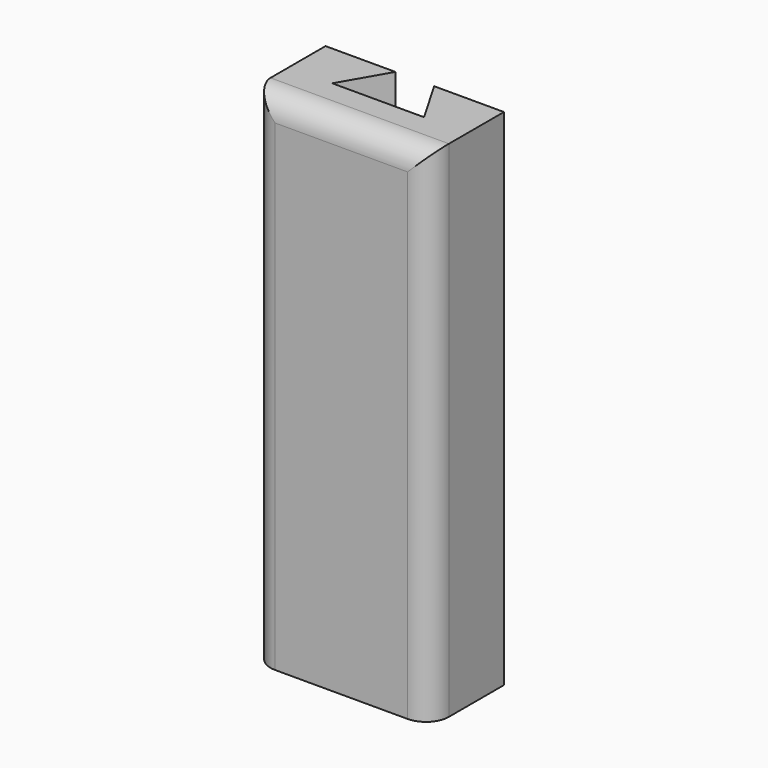
from build123d import *

# Parameters (mm, degrees)
F1_DEPTH    = 279.4
F2_T1_DEPTH = 136.906


# Not quite as in the source:
# - a fillet or chamfer that OpenCascade refuses, or shapes differently, is made with other operations: its cross-section is extruded or revolved along the edge and cut away or added


with BuildPart() as f1:
    # F0 (on Top) → F1 (new body)
    with BuildSketch(Plane.XY):
        with BuildLine():
            Line((49.403, -12.7), (49.403, 25.4))
            Line((49.403, 25.4), (10.7822931626, 25.4))
            Line((10.7822931626, 25.4), (25.44699, 0))
            Line((25.44699, 0), (-25.35301, 0))
            Line((-25.35301, 0), (-10.6883131626, 25.4))
            Line((-10.6883131626, 25.4), (-49.403, 25.4))
            Line((-49.403, 25.4), (-49.403, -12.7))
            ThreePointArc((-49.403, -12.7), (-45.6832561211, -21.6802561211), (-36.703, -25.4))
            Line((-36.703, -25.4), (36.703, -25.4))
            ThreePointArc((36.703, -25.4), (45.6832561211, -21.6802561211), (49.403, -12.7))
        make_face()
    extrude(amount=F1_DEPTH)

    # F2: fillet of radius 12.7 on 1 edges, made by hand

    # F2_s2 → F2_t1 (cut)
    with BuildSketch(Plane.YZ.offset(-68.453)):
        with BuildLine():
            ThreePointArc((-25.4, 266.7), (-21.6802561211, 275.6802561211), (-12.7, 279.4))
            Line((-12.7, 279.4), (-25.4, 279.4))
            Line((-25.4, 279.4), (-25.4, 266.7))
        make_face()
    extrude(amount=F2_T1_DEPTH, mode=Mode.SUBTRACT)


solid = f1.part
